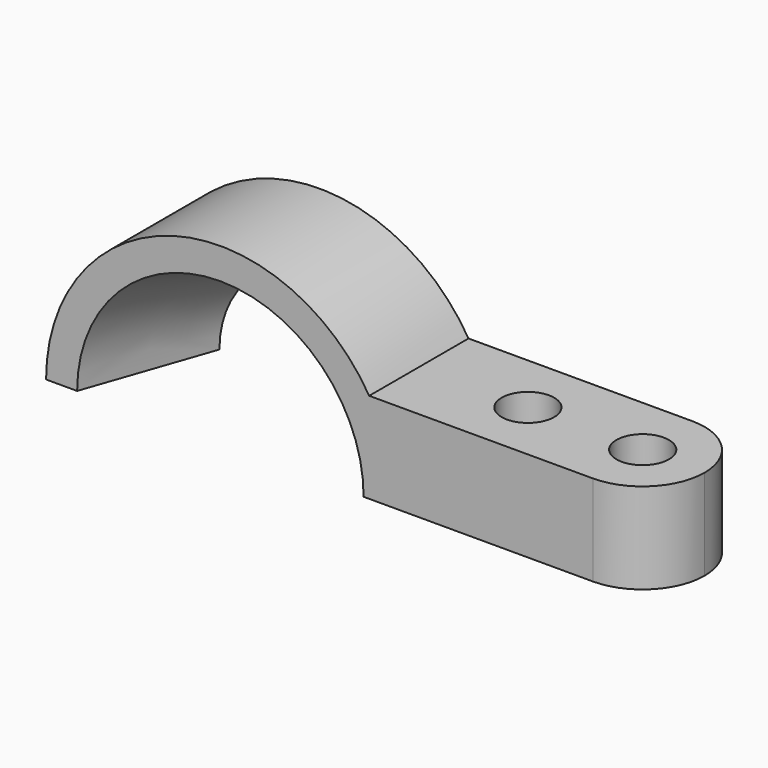
from build123d import *

# Parameters (mm, degrees)
F1_DEPTH = 52
F2_DEPTH = 52
F5_R     = 11
F6_DEPTH = 47.1
F7_R     = 25.99999


# Not quite as in the source:
# - a fillet or chamfer is up to 0.001 mm smaller than in the source, because OpenCascade refuses the exact size


with BuildPart() as f1:
    # F0 (on Front) → F1 (new body)
    with BuildSketch(Plane.XZ):
        with BuildLine():
            Line((81.1170118507, 38), (-38.5532199803, 38))
            ThreePointArc((-38.5532199803, 38), (-120.6178167989, 70.2818364741), (-173.8829881493, 0))
            Line((-173.8829881493, 0), (-160.8829881493, 0))
            ThreePointArc((-160.8829881493, 0), (-100.8829881493, 60), (-40.8829881493, 0))
            Line((-40.8829881493, 0), (-27.8829881493, 0))
            Line((-27.8829881493, 0), (81.1170118507, 0))
            Line((81.1170118507, 0), (81.1170118507, 38))
        make_face()
    extrude(amount=F1_DEPTH)

    # F0 (on Front) → F2 (join)
    with BuildSketch(Plane.XZ):
        with BuildLine():
            ThreePointArc((-40.8829881493, 0), (-100.8829881493, 60), (-160.8829881493, 0))
            Line((-160.8829881493, 0), (-142.8829881493, 0))
            ThreePointArc((-142.8829881493, 0), (-100.8829881493, 42), (-58.8829881493, 0))
            Line((-58.8829881493, 0), (-40.8829881493, 0))
        make_face()
    extrude(amount=F2_DEPTH)

    # F3 (on face) → F4 (revolve, cut)
    with BuildSketch(Plane(origin=(0, 0, 0), x_dir=(1, 0, 0), z_dir=(0, 0, -1))):
        Polygon((-160.8829881493, 52), (-142.8829881493, 0), (-142.8829881493, 52), align=None)
    revolve(axis=Axis((-100.8829881493, -31.7908115685, 0), (0, -1, 0)), mode=Mode.SUBTRACT)

    # F5 (on face) → F6 (cut)
    with BuildSketch(Plane(origin=(0, 0, 0), x_dir=(1, 0, 0), z_dir=(0, 0, -1))):
        with Locations((7.1170118507, 26)):
            Circle(F5_R)
        with Locations((55.1170118507, 25.905281347)):
            Circle(F5_R)
    extrude(amount=-F6_DEPTH, mode=Mode.SUBTRACT)

    # F7 (radius 26 in the source; OpenCascade refuses exactly that, so slightly less here)
    f7_edges = [f1.edges().sort_by_distance(p)[0] for p in [
        (81.117012, -52, 19),
        (81.117012, 0, 19),
    ]]
    fillet(f7_edges, radius=F7_R)


solid = f1.part
